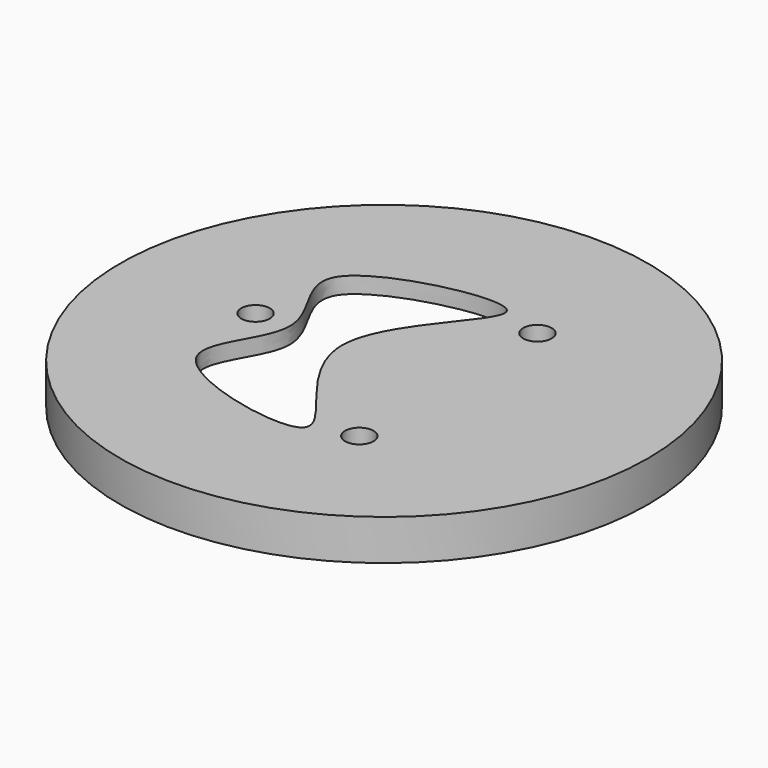
from build123d import *

# Parameters (mm, degrees)
F0_R     = 32.5
F0_R_2   = 1.75
F1_DEPTH = 2
F2_R     = 32.5
F2_R_2   = 31
F3_DEPTH = 3


with BuildPart() as f1:
    # F0 (on Top) → F1 (new body)
    with BuildSketch(Plane.XY):
        with Locations((0.0305813801, -4.44556e-05)):
            Circle(F0_R)
        with Locations((7.944258402, -13.7069351322)):
            Circle(F0_R_2, mode=Mode.SUBTRACT)
        with Locations((-15.7967726636, -4.44556e-05)):
            Circle(F0_R_2, mode=Mode.SUBTRACT)
        with BuildLine():
            add(Edge.make_bspline(
                [(-5.1607941213, -4.44556e-05), (-5.1607941213, 6.8016946043), (13.9227316309, 20.4717509816), (-22.4319309953, 12.4837041278), (-6.7623394337, -4.44556e-05), (-22.4319309953, -12.483793039), (13.9227316309, -20.4718398928), (-5.1607941213, -6.8017835155), (-5.1607941213, -4.44556e-05)],
                knots=[0, 0, 0, 0, 0.177937682, 0.3576170923, 0.5, 0.6423829077, 0.822062318, 1, 1, 1, 1], degree=3))
        make_face(mode=Mode.SUBTRACT)
        with Locations((7.944258402, 13.7068462209)):
            Circle(F0_R_2, mode=Mode.SUBTRACT)
    extrude(amount=F1_DEPTH)

    # F2 (on face) → F3 (join)
    with BuildSketch(Plane(origin=(0, 0, 0), x_dir=(1, 0, 0), z_dir=(0, 0, -1))):
        with Locations((0.0305813801, 4.44556e-05)):
            Circle(F2_R)
        Circle(F2_R_2, mode=Mode.SUBTRACT)
    extrude(amount=F3_DEPTH)


solid = f1.part
